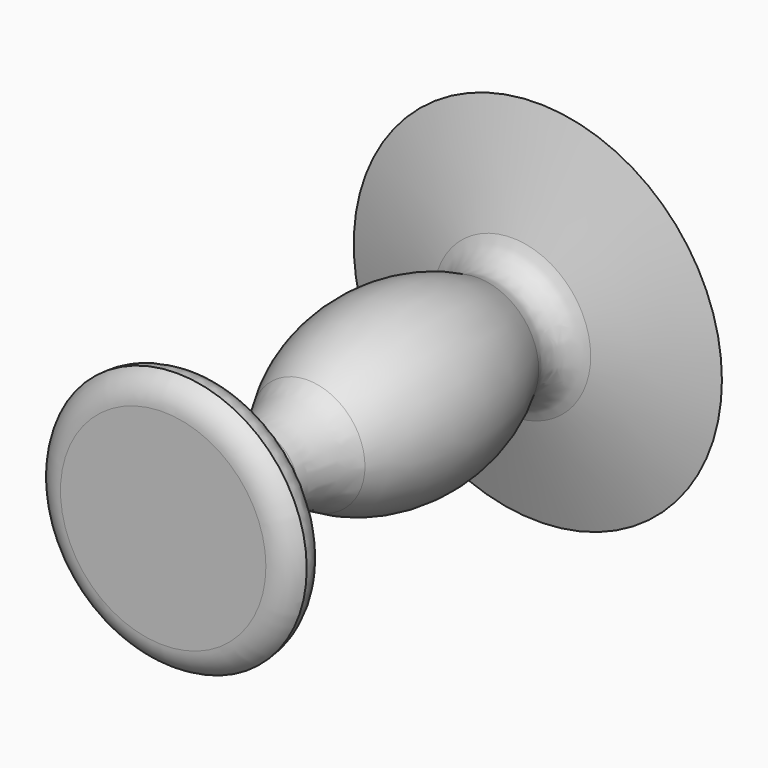
from build123d import *

# Parameters (mm, degrees)
F2_R = 5.08
F3_R = 5.08
F5_R = 20.32
F6_R = 5.08


# Not quite as in the source:
# - a fillet or chamfer that OpenCascade refuses, or shapes differently, is made with other operations: its cross-section is extruded or revolved along the edge and cut away or added


with BuildPart() as f1:
    # F0 (on Top) → F1 (revolve)
    with BuildSketch(Plane.XY):
        with BuildLine():
            Line((0, 41.5879301727), (0, -37.8464572132))
            Line((0, -37.8464572132), (22.0171399415, -37.8464572132))
            Line((22.0171399415, -37.8464572132), (22.0171399415, -31.2269236892))
            Line((22.0171399415, -31.2269236892), (6.7634354346, -26.3342279941))
            Line((6.7634354346, -26.3342279941), (6.7634354346, -11.3683268428))
            ThreePointArc((6.7634354346, -11.3683268428), (14.9158734859, 11.3683268428), (6.7634354346, 34.1049805284))
            Line((6.7634354346, 34.1049805284), (31.2269218266, 41.5879301727))
            Line((31.2269218266, 41.5879301727), (0, 41.5879301727))
        make_face()
    revolve(axis=Axis((0, 1.8707364798, 0), (0, -1, 0)))

    # F2
    f2_edges = [f1.edges().sort_by_distance(p)[0] for p in [
        (-22.01714, -31.226924, 0),
    ]]
    fillet(f2_edges, radius=F2_R)

    # F3
    f3_edges = [f1.edges().sort_by_distance(p)[0] for p in [
        (-6.763435, 34.104981, 0),
    ]]
    fillet(f3_edges, radius=F3_R)

    # F4: fillet of radius 5.08 on 1 edges, made by hand

    # F4_s1 → F4_t2 (revolve, cut)
    with BuildSketch(Plane.XY):
        with BuildLine():
            ThreePointArc((22.0171343212, -34.9324180223), (20.1426258452, -37.0565318577), (17.4220267302, -37.8464572132))
            Line((17.4220267302, -37.8464572132), (22.0171399415, -37.8464572132))
            Line((22.0171399415, -37.8464572132), (22.0171343212, -34.9324180223))
        make_face()
    revolve(axis=Axis((0, -37.8464572132, 0), (0, -1, 0)), mode=Mode.SUBTRACT)

    # F5
    f5_edges = [f1.edges().sort_by_distance(p)[0] for p in [
        (-6.763435, -11.368327, 0),
    ]]
    fillet(f5_edges, radius=F5_R)

    # F6
    f6_edges = [f1.edges().sort_by_distance(p)[0] for p in [
        (-6.763435, -26.334228, 0),
    ]]
    fillet(f6_edges, radius=F6_R)


solid = f1.part
